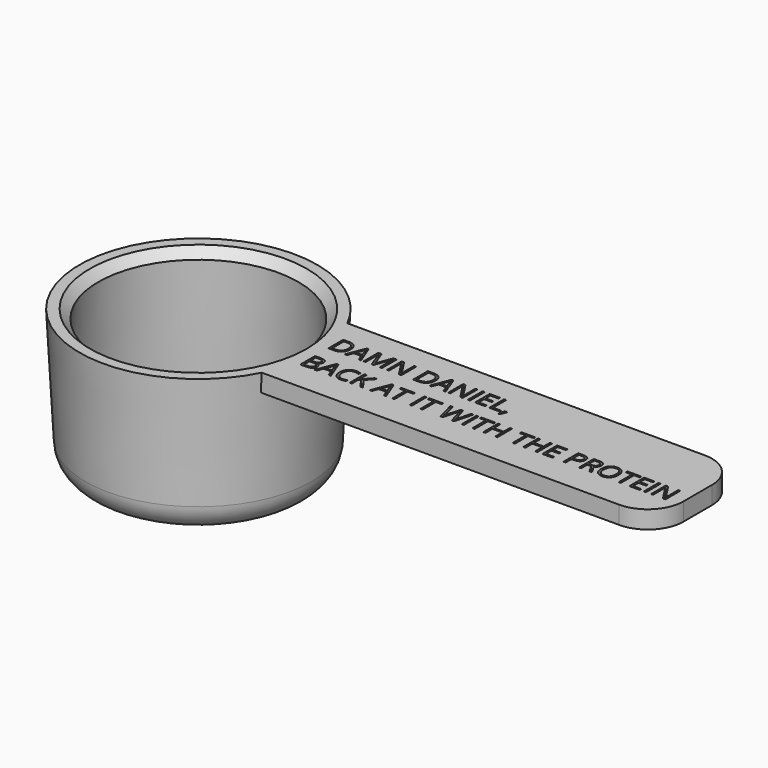
from build123d import *

# Parameters (mm, degrees)
F0_R         = 19.84375
F0_R_2       = 19.05
F1_DEPTH     = 25.4
F1_TAPER     = -3
F2_R         = 19.84375
F3_DEPTH     = 3.175
F7_R         = 6.35
F8_TEXT_SIZE = 4.6001450121
F9_DEPTH     = 0.79375
F10_SIZE     = 1.5875
F11_R        = 5.08


# Not quite as in the source:
# - Text() gives the source's letters only with a copy of the font that has no kerning and outlines rounded to 1/6400 em; it was checked with that copy


with BuildPart() as f1:
    # F0 (on Top) → F1 (new body)
    with BuildSketch(Plane.XY):
        Circle(F0_R)
        Circle(F0_R_2, mode=Mode.SUBTRACT)
    extrude(amount=F1_DEPTH, taper=F1_TAPER)

    # F2 (on Top) → F3 (join)
    with BuildSketch(Plane.XY):
        Circle(F2_R)
    extrude(amount=F3_DEPTH)

    # F5 (on offset) → F6 (join, up to the next surface of F1)
    with BuildSketch(Plane.YZ.offset(88.9)):
        Polygon((9.525, 25.4), (0, 25.4), (-9.525, 25.4), (-9.525, 22.225), (9.525, 22.225), align=None)
    extrude(until=Until.NEXT, dir=(-1, 0, 0))

    # F7
    f7_edges = [f1.edges().sort_by_distance(p)[0] for p in [
        (88.9, -9.525, 23.8125),
        (88.9, 9.525, 23.8125),
    ]]
    fillet(f7_edges, radius=F7_R)

    # F8 (on face) → F9 (cut)
    with BuildSketch(Plane.XY.offset(25.4)):
        with Locations((21.1107313124, 1.9867667877)):
            Text('DAMN DANIEL,', F8_TEXT_SIZE, font='Open Sans', text_align=(TextAlign.LEFT, TextAlign.BOTTOM))
        with Locations((21.1107313124, -4.2694304287)):
            Text('BACK AT IT WITH THE PROTEIN', F8_TEXT_SIZE, font='Open Sans', text_align=(TextAlign.LEFT, TextAlign.BOTTOM))
    extrude(amount=-F9_DEPTH, mode=Mode.SUBTRACT)

    # F10
    f10_edges = [f1.edges().sort_by_distance(p)[0] for p in [
        (-17.718842, 0, 25.4),
    ]]
    chamfer(f10_edges, length=F10_SIZE)

    # F11
    f11_edges = [f1.edges().sort_by_distance(p)[0] for p in [
        (-19.84375, 0, 0),
    ]]
    fillet(f11_edges, radius=F11_R)


solid = f1.part
